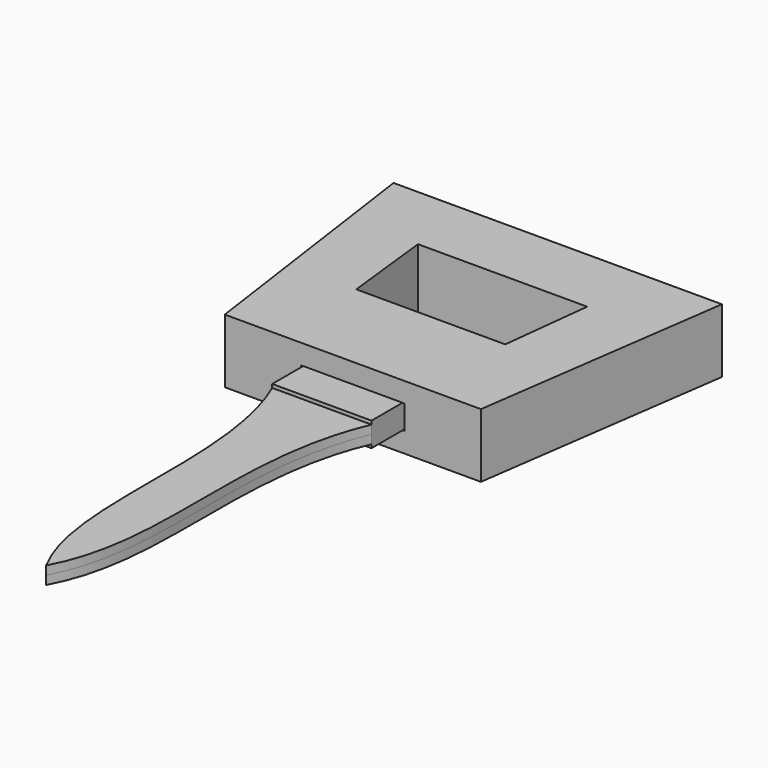
from build123d import *

# Parameters (mm, degrees)
F0_R      = 2.25
F1_DEPTH  = 1.235
F2_DEPTH  = 0.875
F5_DEPTH  = 3.25
F7_DEPTH  = 2.03
F8_R      = 2.0499999718
F9_DEPTH  = 2.03
F10_DEPTH = 4.5


with BuildPart() as f1:
    # F0 (on Top) → F1 (new body, symmetric)
    with BuildSketch(Plane.XY):
        with BuildLine():
            Line((-5.04, 0), (0, 0))
            Line((0, 0), (5.04, 0))
            Line((5.04, 0), (5.04, 5.63))
            Line((5.04, 5.63), (10.4914237453, 5.63))
            ThreePointArc((10.4914237453, 5.63), (11.1606512853, 5.8709517365), (11.5226872593, 6.4832042932))
            Line((11.5226872593, 6.4832042932), (12.4723232041, 11.4635172481))
            ThreePointArc((12.4723232041, 11.4635172481), (12.2499514761, 12.3293840175), (11.4410596901, 12.71))
            Line((11.4410596901, 12.71), (0, 12.71))
            Line((0, 12.71), (-11.4410596901, 12.71))
            ThreePointArc((-11.4410596901, 12.71), (-12.2499514761, 12.3293840175), (-12.4723232041, 11.4635172481))
            Line((-12.4723232041, 11.4635172481), (-11.4888786252, 6.3058967898))
            ThreePointArc((-11.4888786252, 6.3058967898), (-11.2020786705, 5.8208786753), (-10.6719257522, 5.63))
            Line((-10.6719257522, 5.63), (-5.04, 5.63))
            Line((-5.04, 5.63), (-5.04, 0))
        make_face()
        with Locations((7.3813709514, 9.27)):
            Circle(F0_R, mode=Mode.SUBTRACT)
    extrude(amount=F1_DEPTH, both=True)

    # F0 (on Top) → F2 (join, symmetric)
    with BuildSketch(Plane.XY):
        with BuildLine():
            Line((5.04, 0), (0, 0))
            Line((0, 0), (0, -35))
            add(Edge.make_bspline(
                [(0, -35), (5.04, -25.7009714842), (0, -11.7251211777), (5.04, 0)],
                knots=[0, 0, 0, 0, 35.3610180849, 35.3610180849, 35.3610180849, 35.3610180849], degree=3))
        make_face()
        with BuildLine():
            Line((0, -35), (0, 0))
            Line((0, 0), (-5.04, 0))
            add(Edge.make_bspline(
                [(0, -35), (-5.04, -25.7009714842), (0, -11.7251211777), (-5.04, 0)],
                knots=[0, 0, 0, 0, 35.3610180849, 35.3610180849, 35.3610180849, 35.3610180849], degree=3))
        make_face()
    extrude(amount=F2_DEPTH, both=True)


with BuildPart() as f5:
    # F4 (on Top) → F5 (new body, symmetric)
    with BuildSketch(Plane.XY):
        with BuildLine():
            Line((-13, 3.9300001469), (-5.2399998531, 3.9300001469))
            Line((-5.2399998531, 3.9300001469), (-5.2399998531, 5.4300001469))
            Line((-5.2399998531, 5.4300001469), (-10.6719257522, 5.4300001469))
            ThreePointArc((-10.6719257522, 5.4300001469), (-11.3295694887, 5.666781198), (-11.6853389041, 6.2684361434))
            Line((-11.6853389041, 6.2684361434), (-12.668783483, 11.4260566017))
            ThreePointArc((-12.668783483, 11.4260566017), (-12.4040489534, 12.4568748357), (-11.4410596901, 12.9099998531))
            Line((-11.4410596901, 12.9099998531), (11.4410596901, 12.9099998531))
            ThreePointArc((11.4410596901, 12.9099998531), (12.4040489534, 12.4568748357), (12.668783483, 11.4260566017))
            Line((12.668783483, 11.4260566017), (11.7191475382, 6.4457436467))
            ThreePointArc((11.7191475382, 6.4457436467), (11.2881421035, 5.7168542592), (10.4914237453, 5.4300001469))
            Line((10.4914237453, 5.4300001469), (5.2399998531, 5.4300001469))
            Line((5.2399998531, 5.4300001469), (5.2399998531, 3.9300001469))
            Line((5.2399998531, 3.9300001469), (13, 3.9300001469))
            Line((13, 3.9300001469), (16.67, 29.9300001469))
            Line((16.67, 29.9300001469), (0, 29.9300001469))
            Line((0, 29.9300001469), (-16.67, 29.9300001469))
            Line((-16.67, 29.9300001469), (-13, 3.9300001469))
        make_face()
        Polygon((7.56, 13.8200001469), (0, 13.8200001469), (-7.56, 13.8200001469), (-8.59, 22.9300001469), (0, 22.9300001469), (8.59, 22.9300001469), align=None, mode=Mode.SUBTRACT)
    extrude(amount=F5_DEPTH, both=True)

    # F6 (on face) → F7 (join)
    with BuildSketch(Plane.XY.offset(3.25)):
        with BuildLine():
            Line((11.4410596901, 12.9099998531), (-11.4410596901, 12.9099998531))
            ThreePointArc((-11.4410596901, 12.9099998531), (-12.4040489534, 12.4568748357), (-12.668783483, 11.4260566017))
            Line((-12.668783483, 11.4260566017), (-11.6853389041, 6.2684361434))
            ThreePointArc((-11.6853389041, 6.2684361434), (-11.3295694887, 5.666781198), (-10.6719257522, 5.4300001469))
            Line((-10.6719257522, 5.4300001469), (-5.2399998531, 5.4300001469))
            Line((-5.2399998531, 5.4300001469), (-5.2399998531, 3.9300001469))
            Line((-5.2399998531, 3.9300001469), (5.2399998531, 3.9300001469))
            Line((5.2399998531, 3.9300001469), (5.2399998531, 5.4300001469))
            Line((5.2399998531, 5.4300001469), (10.4914237453, 5.4300001469))
            ThreePointArc((10.4914237453, 5.4300001469), (11.2881421035, 5.7168542592), (11.7191475382, 6.4457436467))
            Line((11.7191475382, 6.4457436467), (12.668783483, 11.4260566017))
            ThreePointArc((12.668783483, 11.4260566017), (12.4040489534, 12.4568748357), (11.4410596901, 12.9099998531))
        make_face()
    extrude(amount=-F7_DEPTH)

    # F8 (on face) → F9 (join)
    with BuildSketch(Plane(origin=(0, 0, -3.25), x_dir=(1, 0, 0), z_dir=(0, 0, -1))):
        with BuildLine():
            ThreePointArc((-12.668783483, -11.4260566017), (-12.4040489534, -12.4568748357), (-11.4410596901, -12.9099998531))
            Line((-11.4410596901, -12.9099998531), (11.4410596901, -12.9099998531))
            ThreePointArc((11.4410596901, -12.9099998531), (12.4040489534, -12.4568748357), (12.668783483, -11.4260566017))
            Line((12.668783483, -11.4260566017), (11.7191475382, -6.4457436467))
            ThreePointArc((11.7191475382, -6.4457436467), (11.2881421035, -5.7168542592), (10.4914237453, -5.4300001469))
            Line((10.4914237453, -5.4300001469), (5.2399998531, -5.4300001469))
            Line((5.2399998531, -5.4300001469), (5.2399998531, -3.9300001469))
            Line((5.2399998531, -3.9300001469), (-5.2399998531, -3.9300001469))
            Line((-5.2399998531, -3.9300001469), (-5.2399998531, -5.4300001469))
            Line((-5.2399998531, -5.4300001469), (-10.6719257522, -5.4300001469))
            ThreePointArc((-10.6719257522, -5.4300001469), (-11.3295694887, -5.666781198), (-11.6853389041, -6.2684361434))
            Line((-11.6853389041, -6.2684361434), (-12.668783483, -11.4260566017))
        make_face()
        with Locations((7.3813709514, -9.27)):
            Circle(F8_R, mode=Mode.SUBTRACT)
    extrude(amount=-F9_DEPTH)

    # F8 (on face) → F10 (join)
    with BuildSketch(Plane(origin=(0, 0, -3.25), x_dir=(1, 0, 0), z_dir=(0, 0, -1))):
        with Locations((7.3813709514, -9.27)):
            Circle(F8_R)
    extrude(amount=-F10_DEPTH)


solid = Compound([f1.part, f5.part])
